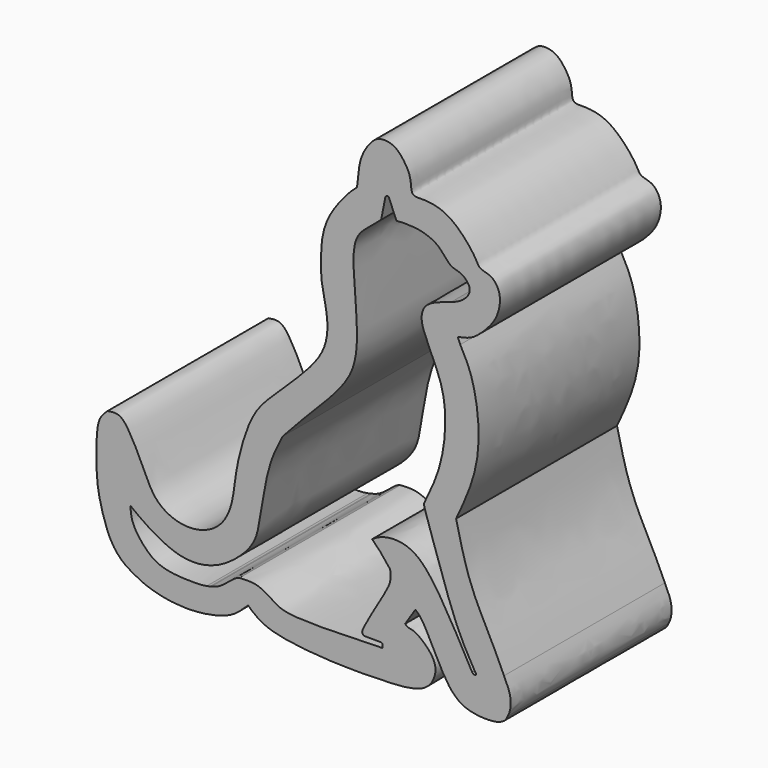
from build123d import *

# Parameters (mm, degrees)
F1_DEPTH = 20


with BuildPart() as f1:
    # F0 (on Front) → F1 (new body)
    with BuildSketch(Plane.XZ):
        with BuildLine():
            add(Edge.make_bspline(
                [(-20.7487847656, 46.1040325463), (-20.3303862754, 45.3399295926), (-19.28563534, 43.4319464275), (-18.4120836912, 36.6303275025), (-20.2447935621, 32.6984309076), (-21.1616884917, 30.7313241065)],
                knots=[0, 0, 0, 0, 0.2502619782, 0.6249100845, 1, 1, 1, 1], degree=3))
            add(Edge.make_bspline(
                [(-20.7487847656, 46.1040325463), (-20.832112059, 46.306459854), (-20.9154393524, 46.5088871618), (-20.9987666458, 46.7113144696)],
                knots=[0, 0, 0, 0, 0.65672085, 0.65672085, 0.65672085, 0.65672085], degree=3))
            add(Edge.make_bspline(
                [(-31.0179907829, 56.5340109169), (-30.9648744466, 57.0992846066), (-30.8607160926, 58.2077567126), (-30.563719391, 59.6727670181), (-29.4102331097, 61.3366997423), (-28.4306155378, 61.6355212683), (-27.2119789694, 61.4263770461), (-26.2908848045, 60.355130686), (-25.5864479717, 59.0864348371), (-25.7013150153, 57.5380427109), (-24.521071204, 57.6407440756), (-23.1122367464, 57.5137758593), (-21.6915658575, 56.9226697311), (-20.1879081771, 55.5128852571), (-19.1819956688, 54.1453522376), (-18.8400482098, 53.2792479551), (-17.4810123693, 53.2211125422), (-16.5676518843, 51.6137269674), (-17.0652941184, 49.6910742329), (-17.8419877787, 48.5931421621), (-19.4350326444, 46.9775813302), (-20.5073184004, 46.7949964649), (-20.9987666458, 46.7113144696)],
                knots=[0, 0, 0, 0, 0.0535142334, 0.1049386095, 0.1623313026, 0.2029684629, 0.2470283969, 0.2955125062, 0.3464492582, 0.3926042226, 0.4317407987, 0.4816279218, 0.5327558165, 0.5926376716, 0.6467690378, 0.6839721864, 0.7284879685, 0.7816317376, 0.8383383699, 0.8873449439, 0.9483681198, 1, 1, 1, 1], degree=3))
            add(Edge.make_bspline(
                [(-55.8274887673, 28.8803216754), (-55.4481147513, 28.9404708949), (-54.6224335956, 29.0713680478), (-53.5452010939, 27.766844997), (-52.1683512696, 24.8178828905), (-51.1215990727, 22.5334444691), (-49.0083031201, 21.3264083443), (-46.6618001584, 21.2444700429), (-44.4505809537, 22.3860014217), (-43.3464604831, 24.7587961987), (-43.1535932955, 27.3995378193), (-42.4429157549, 30.6151230675), (-41.3335746149, 33.4399818324), (-39.7335592777, 35.3520574193), (-35.3413985379, 39.312596738), (-33.9468594003, 41.8792107397), (-33.9132633523, 44.4661929761), (-34.6238780979, 46.9348109475), (-34.6464953873, 49.7012507213), (-34.3258240653, 52.6466349425), (-32.1533168713, 55.5383247345), (-31.3378681642, 56.2534769876), (-31.0179907829, 56.5340109169)],
                knots=[0, 0, 0, 0, 0.0323360437, 0.0703735606, 0.1268466297, 0.1760797335, 0.2224920305, 0.2691496413, 0.3164463015, 0.3650368506, 0.4155709915, 0.4721062517, 0.5248211475, 0.5744347734, 0.6493342676, 0.7023072256, 0.7503369013, 0.7998849262, 0.8509562458, 0.9045972125, 0.9625761688, 1, 1, 1, 1], degree=3))
            add(Edge.make_bspline(
                [(-56.6296465695, 21.0362654179), (-56.8567148857, 21.997683951), (-56.9452028616, 23.8071587367), (-56.958998549, 26.7220144587), (-56.6051108956, 28.1673987142), (-56.0714046211, 28.6574470947), (-55.8274887673, 28.8803216754)],
                knots=[0.6805753879, 0.6805753879, 0.6805753879, 0.6805753879, 0.7775787055, 0.8750068776, 0.9430358524, 1, 1, 1, 1], degree=3))
            add(Edge.make_bspline(
                [(-41.8568353904, 16.3999903506), (-42.1456206316, 16.1307885834), (-42.8166588659, 15.5052430246), (-45.071864052, 14.8778576911), (-46.3063677131, 14.5317571122), (-48.8680971898, 14.5341896941), (-52.101265559, 15.3727480249), (-53.5876667295, 16.3638944998), (-55.5568497498, 17.9929044408), (-56.3895640001, 20.01974389), (-56.6296465695, 21.0362654179)],
                knots=[0, 0, 0, 0, 0.0650598175, 0.1511037288, 0.216775587, 0.3075459623, 0.4121193792, 0.4884679606, 0.5780123966, 0.6805753879, 0.6805753879, 0.6805753879, 0.6805753879], degree=3))
            add(Edge.make_bspline(
                [(-33.5670337081, 14.2084183171), (-35.3062474897, 14.2821540492), (-38.0593911243, 14.552028023), (-40.495375101, 15.2076347559), (-41.4283555671, 16.0247466064), (-41.8568353904, 16.3999903506)],
                knots=[0.6784333616, 0.6784333616, 0.6784333616, 0.6784333616, 0.8166263486, 0.9157868754, 1, 1, 1, 1], degree=3))
            add(Edge.make_bspline(
                [(-31.4194881209, 14.1571559452), (-32.1365515118, 14.1623847378), (-32.8629584574, 14.1785683329), (-33.5670337081, 14.2084183171)],
                knots=[0.622489542, 0.622489542, 0.622489542, 0.622489542, 0.6784333616, 0.6784333616, 0.6784333616, 0.6784333616], degree=3))
            Line((-31.4194881209, 14.1571559452), (-30.3595891519, 14.1571559452))
            add(Edge.make_bspline(
                [(-26.2280292809, 19.8770556599), (-26.1462435368, 19.7879214961), (-25.9647128685, 19.5900803627), (-25.366526783, 19.6378810034), (-24.0113170837, 18.621126751), (-22.9322205591, 17.1282443336), (-23.6028095477, 15.1992166678), (-25.2419621925, 14.3835918255), (-27.4122402143, 14.2153856518), (-29.5122851338, 14.1632147392), (-30.3595891519, 14.1571559452)],
                knots=[0, 0, 0, 0, 0.0379229532, 0.0841733951, 0.166277548, 0.2518007734, 0.3365798004, 0.4191670283, 0.5269190289, 0.5946436392, 0.5946436392, 0.5946436392, 0.5946436392], degree=3))
            Line((-26.2280292809, 19.8770556599), (-25.2116527408, 21.4492641389))
            add(Edge.make_bspline(
                [(-24.2429170758, 20.2264357358), (-24.4292858715, 20.5303672934), (-24.757029312, 21.0648536269), (-25.0746462434, 21.3334171885), (-25.2116527408, 21.4492641389)],
                knots=[0, 0, 0, 0, 0.5686423365, 1, 1, 1, 1], degree=3))
            add(Edge.make_bspline(
                [(-21.5114019811, 15.4145238921), (-22.1834113624, 16.1377463355), (-23.3761446891, 18.5598980326), (-23.9861726894, 19.7327949525), (-24.2429170758, 20.2264357358)],
                knots=[0.6969094598, 0.6969094598, 0.6969094598, 0.6969094598, 0.8724373394, 1, 1, 1, 1], degree=3))
            add(Edge.make_bspline(
                [(-21.5114019811, 15.4145238921), (-21.4570188523, 15.3597391252), (-21.4026357234, 15.3049543582), (-21.3474047999, 15.2507544558)],
                knots=[0, 0, 0, 0, 0.03867594, 0.03867594, 0.03867594, 0.03867594], degree=3))
            add(Edge.make_bspline(
                [(-16.0324927419, 15.0969056413), (-16.2580678871, 14.7175649662), (-17.0053841987, 14.2040613308), (-18.6732979158, 14.2091952737), (-20.1398294643, 14.5614082384), (-20.9603259438, 14.8933560009), (-21.3474047999, 15.2507544558)],
                knots=[0.2460810052, 0.2460810052, 0.2460810052, 0.2460810052, 0.3491172355, 0.4665634461, 0.5811990996, 0.6826058072, 0.6826058072, 0.6826058072, 0.6826058072], degree=3))
            add(Edge.make_bspline(
                [(-16.3964722306, 18.5242276639), (-16.117109962, 17.9476686591), (-15.5745773683, 16.827968229), (-15.7711620256, 15.5363750264), (-16.0324927419, 15.0969056413)],
                knots=[0, 0, 0, 0, 0.1267126596, 0.2460810052, 0.2460810052, 0.2460810052, 0.2460810052], degree=3))
            add(Edge.make_bspline(
                [(-16.3964722306, 18.5242276639), (-16.8194092062, 19.447542096), (-17.7463781461, 21.4712095682), (-19.9262523685, 25.4785396975), (-20.7369751703, 28.9255427547), (-21.1616884917, 30.7313241065)],
                knots=[0, 0, 0, 0, 0.2854714806, 0.6256799735, 1, 1, 1, 1], degree=3))
        make_face()
        with BuildLine():
            add(Edge.make_bspline(
                [(-38.4316630661, 32.3070697486), (-38.787613223, 31.6073751487), (-39.5328846714, 30.1423879929), (-40.2117006876, 27.4814020453), (-40.7341829263, 23.7285908482), (-41.2735565273, 21.8096847799), (-43.4041728597, 19.6453127354), (-45.9825109703, 18.3436355754), (-48.9766519488, 18.3929871464), (-51.954069101, 20.0945764095), (-53.0730808934, 20.957499025), (-53.5602457821, 21.33317478)],
                knots=[0, 0, 0, 0, 0.1031925341, 0.2160596023, 0.3458453271, 0.4405113384, 0.5543241777, 0.6677461712, 0.781890915, 0.9050456046, 1, 1, 1, 1], degree=3))
            add(Edge.make_bspline(
                [(-38.4316630661, 32.3070697486), (-38.0281427128, 32.7620371618), (-37.0542220616, 33.8601283937), (-34.2044762766, 36.6569980992), (-32.151144328, 38.9997659752), (-31.1913969222, 40.9273322513), (-30.8687323947, 43.9537013314), (-31.4299236985, 48.8608141493), (-31.3625693365, 52.1887657958), (-29.8552389788, 53.4188783759), (-29.0250026537, 54.1283648868), (-28.6172647029, 54.476801306)],
                knots=[0, 0, 0, 0, 0.0949138172, 0.2290802094, 0.3476169046, 0.4421701159, 0.5571862518, 0.7082250492, 0.8268529619, 0.9149656362, 1, 1, 1, 1], degree=3))
            Line((-28.6172647029, 54.476801306), (-28.19892826, 56.5980450867))
            ThreePointArc((-28.19892826, 56.5980450867), (-28.0593765242, 56.7511515184), (-27.8590243823, 56.6984705388))
            Line((-27.8590243823, 56.6984705388), (-27.0926989615, 54.8927225173))
            add(Edge.make_bspline(
                [(-21.6667801142, 49.5260991156), (-21.2800939418, 49.6694728072), (-20.4961968386, 49.960122511), (-19.4319769369, 51.211270264), (-20.5806460366, 52.5095551917), (-21.8060870275, 52.5029092101), (-22.7965234524, 54.243806652), (-25.0427924808, 54.9823622196), (-26.4213925163, 54.9220778613), (-27.0926989615, 54.8927225173)],
                knots=[0, 0, 0, 0, 0.1281974702, 0.2598841974, 0.3926604126, 0.5129371219, 0.6653859691, 0.8370603875, 1, 1, 1, 1], degree=3))
            add(Edge.make_bspline(
                [(-24.3430305272, 31.0551617295), (-23.7540348779, 32.272455353), (-22.5541134177, 34.7523662727), (-22.062454118, 39.3023120815), (-22.6379130941, 42.5371989194), (-24.4107201365, 45.8833660311), (-24.7013621135, 47.4175767754), (-24.1472826268, 48.7525720618), (-22.59215326, 49.2375280863), (-21.6667801142, 49.5260991156)],
                knots=[0, 0, 0, 0, 0.1718842225, 0.3501682355, 0.5061378796, 0.6689010582, 0.7717763593, 0.8641964888, 1, 1, 1, 1], degree=3))
            add(Edge.make_bspline(
                [(-19.3159710616, 18.0031750351), (-19.9049136192, 19.0221989297), (-21.2681302703, 21.3809185078), (-23.1836058674, 27.3519502792), (-24.3629778292, 30.6638019753), (-24.3467341053, 30.9824987002), (-24.3430305272, 31.0551617295)],
                knots=[0, 0, 0, 0, 0.2851847094, 0.6601128404, 0.92250554, 1, 1, 1, 1], degree=3))
            add(Edge.make_bspline(
                [(-19.5520427078, 17.7765469998), (-19.4974018907, 17.7239619053), (-19.3907813166, 17.6213526607), (-19.0627144504, 17.6712339879), (-19.2247656463, 17.8836329591), (-19.3159710616, 18.0031750351)],
                knots=[0, 0, 0, 0, 0.31486324, 0.614392338, 1, 1, 1, 1], degree=3))
            add(Edge.make_bspline(
                [(-29.5156072825, 26.2166075408), (-29.2794558859, 26.3702154382), (-28.7510224742, 26.7139421592), (-27.3759014589, 27.0011909743), (-25.8628232557, 26.7773134652), (-23.6521619439, 25.3363888928), (-21.18396965, 20.7855106307), (-19.5520427078, 17.7765469998)],
                knots=[0, 0, 0, 0, 0.1208996361, 0.2705358007, 0.4239578557, 0.6191306904, 1, 1, 1, 1], degree=3))
            add(Edge.make_bspline(
                [(-27.7217533439, 24.1623837501), (-28.1212664349, 24.6684329563), (-28.8103627935, 25.541287121), (-29.3069312274, 26.0167857722), (-29.5156072825, 26.2166075408)],
                knots=[0, 0, 0, 0, 0.5797637529, 1, 1, 1, 1], degree=3))
            add(Edge.make_bspline(
                [(-30.2724037319, 17.4852889031), (-30.3533347919, 17.5254686643), (-30.5222812548, 17.6093453432), (-30.4918371637, 17.9833782238), (-30.0719211893, 18.7727874381), (-28.9541595874, 20.7571792697), (-27.7229642372, 22.7356672715), (-27.6639890575, 23.5366461821), (-27.7031893951, 23.9612878674), (-27.7217533439, 24.1623837501)],
                knots=[0, 0, 0, 0, 0.074653362, 0.1558415456, 0.2933080614, 0.5252806576, 0.7545360943, 0.8837566295, 1, 1, 1, 1], degree=3))
            add(Edge.make_bspline(
                [(-28.5034030676, 17.0203652233), (-28.4727033297, 17.1734470604), (-28.4077025034, 17.4975685868), (-29.057037387, 17.4796026733), (-29.8065621175, 17.4831094101), (-30.2724037319, 17.4852889031)],
                knots=[0, 0, 0, 0, 0.2530323645, 0.5357476611, 1, 1, 1, 1], degree=3))
            add(Edge.make_bspline(
                [(-28.5034030676, 17.0203652233), (-32.3234946028, 16.8915965478), (-37.6340461121, 16.7125870456), (-39.1123516704, 17.4274657192), (-40.1755302254, 18.1863361205), (-41.326562361, 18.6188056298), (-42.2399300621, 18.5582096478), (-42.7117981017, 18.526904285)],
                knots=[0, 0, 0, 0, 0.4007144523, 0.557058573, 0.701666425, 0.8458735962, 1, 1, 1, 1], degree=3))
            add(Edge.make_bspline(
                [(-45.5234933543, 16.8591268329), (-45.2896875752, 16.9174889426), (-44.6368275844, 17.1278035198), (-43.6816191999, 17.9234751873), (-43.132809663, 18.3891088567), (-42.8389775629, 18.4852789475), (-42.7117981017, 18.526904285)],
                knots=[0.1142431913, 0.1142431913, 0.1142431913, 0.1142431913, 0.2908301862, 0.6068321923, 0.8298250261, 1, 1, 1, 1], degree=3))
            add(Edge.make_bspline(
                [(-45.6433745919, 16.8305592422), (-45.6038950049, 16.8397206685), (-45.5639076609, 16.8492542278), (-45.5234933543, 16.8591268329)],
                knots=[0.6772499898, 0.6772499898, 0.6772499898, 0.6772499898, 0.6856185308, 0.6856185308, 0.6856185308, 0.6856185308], degree=3))
            add(Edge.make_bspline(
                [(-45.9770783782, 16.7601127177), (-45.8716305697, 16.7797994172), (-45.7597069364, 16.8035637671), (-45.6433745919, 16.8305592422)],
                knots=[0.6525908667, 0.6525908667, 0.6525908667, 0.6525908667, 0.6772499898, 0.6772499898, 0.6772499898, 0.6772499898], degree=3))
            add(Edge.make_bspline(
                [(-53.5602457821, 21.33317478), (-53.5275000285, 20.8858182837), (-53.456674732, 19.9182376693), (-52.3715321356, 18.3186243864), (-50.6345346652, 16.7200607918), (-47.2965162079, 16.6541107546), (-46.4411221179, 16.6734775398), (-45.9770783782, 16.7601127177)],
                knots=[0, 0, 0, 0, 0.109033279, 0.2358264337, 0.3784731562, 0.5440735645, 0.6525908667, 0.6525908667, 0.6525908667, 0.6525908667], degree=3))
        make_face(mode=Mode.SUBTRACT)
        with BuildLine():
            add(Edge.make_bspline(
                [(-18.0320851505, 14.1571559452), (-17.6403274955, 14.1631609), (-16.9815269838, 14.2283270543), (-16.2381293963, 14.6145982321), (-16.0956973772, 14.9486632767), (-16.0324927419, 15.0969056413)],
                knots=[0.5627914432, 0.5627914432, 0.5627914432, 0.5627914432, 0.7361679796, 0.8829237504, 1, 1, 1, 1], degree=3))
            add(Edge.make_bspline(
                [(-16.0324927419, 15.0969056413), (-16.2580678871, 14.7175649662), (-17.0053841987, 14.2040613308), (-18.6732979158, 14.2091952737), (-20.1398294643, 14.5614082384), (-20.9603259438, 14.8933560009), (-21.3474047999, 15.2507544558)],
                knots=[0.2460810052, 0.2460810052, 0.2460810052, 0.2460810052, 0.3491172355, 0.4665634461, 0.5811990996, 0.6826058072, 0.6826058072, 0.6826058072, 0.6826058072], degree=3))
            add(Edge.make_bspline(
                [(-21.3474047999, 15.2507544558), (-21.1604217834, 15.0672619376), (-20.6728491649, 14.6290436116), (-19.5417962952, 14.2402668664), (-18.6532022738, 14.1630875988), (-18.2681223709, 14.1571559452)],
                knots=[0.03867594, 0.03867594, 0.03867594, 0.03867594, 0.1696124419, 0.3632364931, 0.5285271602, 0.5285271602, 0.5285271602, 0.5285271602], degree=3))
            Line((-18.2681223709, 14.1571559452), (-18.0320851505, 14.1571559452))
        make_face()
        with BuildLine():
            add(Edge.make_bspline(
                [(-41.8568353904, 16.3999903506), (-42.1456206316, 16.1307885834), (-42.8166588659, 15.5052430246), (-45.071864052, 14.8778576911), (-46.3063677131, 14.5317571122), (-48.8680971898, 14.5341896941), (-52.101265559, 15.3727480249), (-53.5876667295, 16.3638944998), (-55.5568497498, 17.9929044408), (-56.3895640001, 20.01974389), (-56.6296465695, 21.0362654179)],
                knots=[0, 0, 0, 0, 0.0650598175, 0.1511037288, 0.216775587, 0.3075459623, 0.4121193792, 0.4884679606, 0.5780123966, 0.6805753879, 0.6805753879, 0.6805753879, 0.6805753879], degree=3))
            add(Edge.make_bspline(
                [(-56.6296465695, 21.0362654179), (-56.4890989004, 20.2997960238), (-56.2041033451, 19.4739372016), (-55.6858486145, 17.7995716288), (-54.4551002842, 16.0756422454), (-53.2276345192, 15.4562696348), (-52.6236931649, 15.1591578508)],
                knots=[0, 0, 0, 0, 0.2385855592, 0.4744125714, 0.7385609639, 1, 1, 1, 1], degree=3))
            add(Edge.make_bspline(
                [(-48.0707209539, 14.1571559452), (-48.958031374, 14.1685917112), (-50.5444395864, 14.3634058238), (-52.052806606, 14.8685211605), (-52.6236931649, 15.1591578508)],
                knots=[0.4985836744, 0.4985836744, 0.4985836744, 0.4985836744, 0.6667451418, 0.7975818843, 0.7975818843, 0.7975818843, 0.7975818843], degree=3))
            Line((-48.0707209539, 14.1571559452), (-47.7607548237, 14.1571559452))
            add(Edge.make_bspline(
                [(-41.8568353904, 16.3999903506), (-42.3047837772, 15.9607076096), (-43.2112203415, 15.0718298385), (-45.0928687784, 14.3973445873), (-46.8175939501, 14.1693326421), (-47.7607548237, 14.1571559452)],
                knots=[0, 0, 0, 0, 0.1482248179, 0.2999284062, 0.4789866672, 0.4789866672, 0.4789866672, 0.4789866672], degree=3))
        make_face()
        with BuildLine():
            add(Edge.make_bspline(
                [(-45.9770783782, 16.7601127177), (-45.8658569179, 16.782648325), (-45.7546354576, 16.8051839322), (-45.6433745919, 16.8305592422)],
                knots=[0, 0, 0, 0, 0.0840574475, 0.0840574475, 0.0840574475, 0.0840574475], degree=3))
            add(Edge.make_bspline(
                [(-45.9770783782, 16.7601127177), (-45.8716305697, 16.7797994172), (-45.7597069364, 16.8035637671), (-45.6433745919, 16.8305592422)],
                knots=[0.6525908667, 0.6525908667, 0.6525908667, 0.6525908667, 0.6772499898, 0.6772499898, 0.6772499898, 0.6772499898], degree=3))
        make_face()
    extrude(amount=F1_DEPTH)


solid = f1.part
